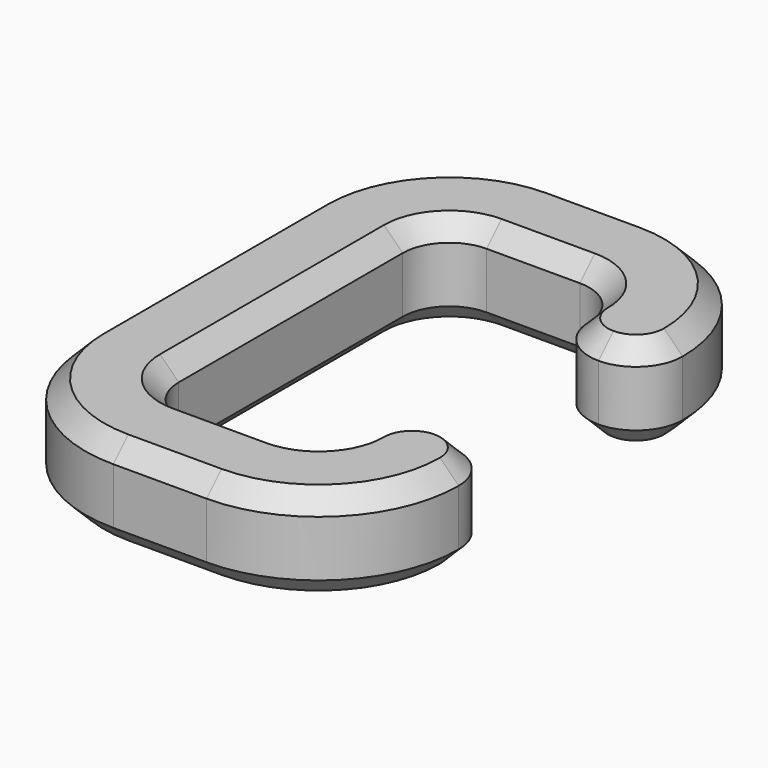
from build123d import *

# Parameters (mm, degrees)
F0_W         = 10
F0_H         = 10
F1_DEPTH     = 10
F2_R         = 4.99999
F3_R         = 15
F4_T1_DEPTH  = 30.00002
F4_T3_DEPTH  = 10
F4_T5_DEPTH  = 1e-05
F4_T7_DEPTH  = 2e-05
F4_T9_DEPTH  = 2e-05
F4_T11_DEPTH = 10.00002
F4_T13_DEPTH = 2e-05
F4_T15_DEPTH = 1e-05
F4_T17_DEPTH = 30
F4_T20_ANGLE = 90
F4_T22_ANGLE = 90
F4_T24_ANGLE = 90
F4_T26_ANGLE = 90
F4_T28_ANGLE = 90
F4_T30_ANGLE = 90
F4_T32_ANGLE = 90
F4_T34_ANGLE = 90
F4_T36_ANGLE = 90
F4_T38_ANGLE = 90
F4_T40_ANGLE = 90
F4_T42_ANGLE = 90
F4_T44_ANGLE = 90
F4_T46_ANGLE = 90
F4_T48_ANGLE = 90
F4_T50_ANGLE = 90
F4_T52_ANGLE = 90
F4_T54_ANGLE = 90
F4_T56_ANGLE = 90
F4_T58_ANGLE = 90
F4_T60_ANGLE = 90
F4_T62_ANGLE = 90
F4_T64_ANGLE = 90
F4_T66_ANGLE = 90


# Not quite as in the source:
# - a fillet or chamfer that OpenCascade refuses, or shapes differently, is made with other operations: its cross-section is extruded or revolved along the edge and cut away or added
# - a fillet or chamfer is up to 0.001 mm smaller than in the source, because OpenCascade refuses the exact size


with BuildPart() as f1:
    # F0 (on Top) → F1 (new body)
    with BuildSketch(Plane.XY):
        Polygon((-10.4597477218, 27.6766866998), (-10.4597477218, 17.6766866998), (-0.4597477218, 17.6766866998), (-0.4597477218, 37.6766866998), (-10.4597477218, 37.6766866998), align=None)
        Polygon((-30.4597477218, 27.6766866998), (-10.4597477218, 27.6766866998), (-10.4597477218, 37.6766866998), (-40.4597477218, 37.6766866998), (-40.4597477218, 27.6766866998), align=None)
        Polygon((-30.4597477218, -12.3233133002), (-30.4597477218, 27.6766866998), (-40.4597477218, 27.6766866998), (-40.4597477218, -22.3233133002), (-30.4597477218, -22.3233133002), align=None)
        Polygon((-10.4597477218, -12.3233133002), (-30.4597477218, -12.3233133002), (-30.4597477218, -22.3233133002), (-0.4597477218, -22.3233133002), (-0.4597477218, -12.3233133002), align=None)
        with Locations((-5.4597477218, -7.3233133002)):
            Rectangle(F0_W, F0_H)
    extrude(amount=F1_DEPTH)

    # F2 (radius 5 in the source; OpenCascade refuses exactly that, so slightly less here)
    f2_edges = [f1.edges().sort_by_distance(p)[0] for p in [
        (-0.459748, 17.676687, 5),
        (-10.459748, 17.676687, 5),
        (-10.459748, 27.676687, 5),
        (-30.459748, 27.676687, 5),
        (-30.459748, -12.323313, 5),
        (-10.459748, -12.323313, 5),
        (-10.459748, -2.323313, 5),
        (-0.459748, -2.323313, 5),
    ]]
    fillet(f2_edges, radius=F2_R)

    # F3
    f3_edges = [f1.edges().sort_by_distance(p)[0] for p in [
        (-0.459748, 37.676687, 5),
        (-40.459748, 37.676687, 5),
        (-0.459748, -22.323313, 5),
        (-40.459748, -22.323313, 5),
    ]]
    fillet(f3_edges, radius=F3_R)

    # F4: chamfer of 2 on 2 edges, made by hand

    # F4_s2 → F4_t1 (cut)
    with BuildSketch(Plane.XZ.offset(-22.6766966998)):
        Polygon((-30.4597477218, 8), (-32.4597477218, 10), (-30.4597477218, 10), align=None)
        Polygon((-32.4597477218, 0), (-30.4597477218, 2), (-30.4597477218, 0), align=None)
    extrude(amount=F4_T1_DEPTH, mode=Mode.SUBTRACT)

    # F4_s4 → F4_t3 (cut)
    with BuildSketch(Plane.YZ.offset(-25.4597477218)):
        Polygon((-20.3233133002, 0), (-22.3233133002, 2), (-22.3233133002, 0), align=None)
        Polygon((35.6766866998, 0), (37.6766866998, 2), (37.6766866998, 0), align=None)
        Polygon((37.6766866998, 8), (35.6766866998, 10), (37.6766866998, 10), align=None)
        Polygon((-22.3233133002, 8), (-20.3233133002, 10), (-22.3233133002, 10), align=None)
    extrude(amount=F4_T3_DEPTH, mode=Mode.SUBTRACT)

    # F4_s6 → F4_t5 (cut)
    with BuildSketch(Plane.XZ.offset(7.3233033002)):
        Polygon((-2.4597477218, 0), (-0.4597477218, 2), (-0.4597477218, 0), align=None)
        Polygon((-0.4597477218, 8), (-2.4597477218, 10), (-0.4597477218, 10), align=None)
    extrude(amount=F4_T5_DEPTH, mode=Mode.SUBTRACT)

    # F4_s8 → F4_t7 (cut)
    with BuildSketch(Plane.YZ.offset(-5.4597577218)):
        Polygon((-4.3233133002, 0), (-2.3233133002, 2), (-2.3233133002, 0), align=None)
        Polygon((19.6766866998, 0), (17.6766866998, 2), (17.6766866998, 0), align=None)
        Polygon((17.6766866998, 8), (19.6766866998, 10), (17.6766866998, 10), align=None)
        Polygon((-2.3233133002, 8), (-4.3233133002, 10), (-2.3233133002, 10), align=None)
    extrude(amount=F4_T7_DEPTH, mode=Mode.SUBTRACT)

    # F4_s10 → F4_t9 (cut)
    with BuildSketch(Plane.XZ.offset(7.3233033002)):
        Polygon((-8.4597477218, 0), (-10.4597477218, 2), (-10.4597477218, 0), align=None)
        Polygon((-10.4597477218, 8), (-8.4597477218, 10), (-10.4597477218, 10), align=None)
    extrude(amount=F4_T9_DEPTH, mode=Mode.SUBTRACT)

    # F4_s12 → F4_t11 (cut)
    with BuildSketch(Plane.YZ.offset(-25.4597577218)):
        Polygon((-14.3233133002, 0), (-12.3233133002, 2), (-12.3233133002, 0), align=None)
        Polygon((29.6766866998, 0), (27.6766866998, 2), (27.6766866998, 0), align=None)
        Polygon((27.6766866998, 8), (29.6766866998, 10), (27.6766866998, 10), align=None)
        Polygon((-12.3233133002, 8), (-14.3233133002, 10), (-12.3233133002, 10), align=None)
    extrude(amount=F4_T11_DEPTH, mode=Mode.SUBTRACT)

    # F4_s14 → F4_t13 (cut)
    with BuildSketch(Plane.XZ.offset(-22.6766966998)):
        Polygon((-8.4597477218, 0), (-10.4597477218, 2), (-10.4597477218, 0), align=None)
        Polygon((-10.4597477218, 8), (-8.4597477218, 10), (-10.4597477218, 10), align=None)
    extrude(amount=F4_T13_DEPTH, mode=Mode.SUBTRACT)

    # F4_s16 → F4_t15 (cut)
    with BuildSketch(Plane.XZ.offset(-22.6766866998)):
        Polygon((-2.4597477218, 0), (-0.4597477218, 2), (-0.4597477218, 0), align=None)
        Polygon((-0.4597477218, 8), (-2.4597477218, 10), (-0.4597477218, 10), align=None)
    extrude(amount=F4_T15_DEPTH, mode=Mode.SUBTRACT)

    # F4_s18 → F4_t17 (cut)
    with BuildSketch(Plane.XZ.offset(-22.6766866998)):
        Polygon((-38.4597477218, 0), (-40.4597477218, 2), (-40.4597477218, 0), align=None)
        Polygon((-40.4597477218, 8), (-38.4597477218, 10), (-40.4597477218, 10), align=None)
    extrude(amount=F4_T17_DEPTH, mode=Mode.SUBTRACT)

    # F4_s19 → F4_t20 (revolve, cut)
    with BuildSketch(Plane.YZ.offset(-15.4597477218)):
        Polygon((-20.3233133002, 0), (-22.3233133002, 2), (-22.3233133002, 0), align=None)
    revolve(axis=Axis((-15.4597477218, -7.3233133002, 0), (0, 0, 1)), revolution_arc=F4_T20_ANGLE, mode=Mode.SUBTRACT)

    # F4_s21 → F4_t22 (revolve, cut)
    with BuildSketch(Plane.XZ.offset(7.3233033002)):
        Polygon((-2.4597477218, 0), (-0.4597477218, 2), (-0.4597477218, 0), align=None)
    revolve(axis=Axis((-5.4597377218, -7.3233033002, 0), (0, 0, 1)), revolution_arc=F4_T22_ANGLE, mode=Mode.SUBTRACT)

    # F4_s23 → F4_t24 (revolve, cut)
    with BuildSketch(Plane.YZ.offset(-5.4597577218)):
        Polygon((-4.3233133002, 0), (-2.3233133002, 2), (-2.3233133002, 0), align=None)
    revolve(axis=Axis((-5.4597577218, -7.3233033002, 0), (0, 0, 1)), revolution_arc=F4_T24_ANGLE, mode=Mode.SUBTRACT)

    # F4_s25 → F4_t26 (revolve, cut)
    with BuildSketch(Plane.XZ.offset(7.3233233002)):
        Polygon((-8.4597477218, 0), (-10.4597477218, 2), (-10.4597477218, 0), align=None)
    revolve(axis=Axis((-15.4597377218, -7.3233233002, 0), (0, 0, -1)), revolution_arc=F4_T26_ANGLE, mode=Mode.SUBTRACT)

    # F4_s27 → F4_t28 (revolve, cut)
    with BuildSketch(Plane.YZ.offset(-25.4597577218)):
        Polygon((-14.3233133002, 0), (-12.3233133002, 2), (-12.3233133002, 0), align=None)
    revolve(axis=Axis((-25.4597577218, -7.3233233002, 0), (0, 0, -1)), revolution_arc=F4_T28_ANGLE, mode=Mode.SUBTRACT)

    # F4_s29 → F4_t30 (revolve, cut)
    with BuildSketch(Plane.XZ.offset(-22.6766966998)):
        Polygon((-32.4597477218, 0), (-30.4597477218, 2), (-30.4597477218, 0), align=None)
    revolve(axis=Axis((-25.4597577218, 22.6766966998, 0), (0, 0, -1)), revolution_arc=F4_T30_ANGLE, mode=Mode.SUBTRACT)

    # F4_s31 → F4_t32 (revolve, cut)
    with BuildSketch(Plane.XZ.offset(-22.6766966998)):
        Polygon((-8.4597477218, 0), (-10.4597477218, 2), (-10.4597477218, 0), align=None)
    revolve(axis=Axis((-15.4597377218, 22.6766966998, 0), (0, 0, 1)), revolution_arc=F4_T32_ANGLE, mode=Mode.SUBTRACT)

    # F4_s33 → F4_t34 (revolve, cut)
    with BuildSketch(Plane.XZ.offset(-22.6766766998)):
        Polygon((-8.4597477218, 0), (-10.4597477218, 2), (-10.4597477218, 0), align=None)
    revolve(axis=Axis((-5.4597577218, 22.6766766998, 0), (0, 0, 1)), revolution_arc=F4_T34_ANGLE, mode=Mode.SUBTRACT)

    # F4_s35 → F4_t36 (revolve, cut)
    with BuildSketch(Plane.YZ.offset(-5.4597377218)):
        Polygon((19.6766866998, 0), (17.6766866998, 2), (17.6766866998, 0), align=None)
    revolve(axis=Axis((-5.4597377218, 22.6766766998, 0), (0, 0, 1)), revolution_arc=F4_T36_ANGLE, mode=Mode.SUBTRACT)

    # F4_s37 → F4_t38 (revolve, cut)
    with BuildSketch(Plane.XZ.offset(-22.6766866998)):
        Polygon((-2.4597477218, 0), (-0.4597477218, 2), (-0.4597477218, 0), align=None)
    revolve(axis=Axis((-15.4597477218, 22.6766866998, 0), (0, 0, 1)), revolution_arc=F4_T38_ANGLE, mode=Mode.SUBTRACT)

    # F4_s39 → F4_t40 (revolve, cut)
    with BuildSketch(Plane.YZ.offset(-25.4597477218)):
        Polygon((35.6766866998, 0), (37.6766866998, 2), (37.6766866998, 0), align=None)
    revolve(axis=Axis((-25.4597477218, 22.6766866998, 0), (0, 0, 1)), revolution_arc=F4_T40_ANGLE, mode=Mode.SUBTRACT)

    # F4_s41 → F4_t42 (revolve, cut)
    with BuildSketch(Plane.XZ.offset(7.3233133002)):
        Polygon((-38.4597477218, 0), (-40.4597477218, 2), (-40.4597477218, 0), align=None)
    revolve(axis=Axis((-25.4597477218, -7.3233133002, 0), (0, 0, 1)), revolution_arc=F4_T42_ANGLE, mode=Mode.SUBTRACT)

    # F4_s43 → F4_t44 (revolve, cut)
    with BuildSketch(Plane.YZ.offset(-25.4597577218)):
        Polygon((-12.3233133002, 8), (-14.3233133002, 10), (-12.3233133002, 10), align=None)
    revolve(axis=Axis((-25.4597577218, -7.3233233002, 10), (0, 0, -1)), revolution_arc=F4_T44_ANGLE, mode=Mode.SUBTRACT)

    # F4_s45 → F4_t46 (revolve, cut)
    with BuildSketch(Plane.XZ.offset(-22.6766966998)):
        Polygon((-30.4597477218, 8), (-32.4597477218, 10), (-30.4597477218, 10), align=None)
    revolve(axis=Axis((-25.4597577218, 22.6766966998, 10), (0, 0, -1)), revolution_arc=F4_T46_ANGLE, mode=Mode.SUBTRACT)

    # F4_s47 → F4_t48 (revolve, cut)
    with BuildSketch(Plane.XZ.offset(-22.6766966998)):
        Polygon((-10.4597477218, 8), (-8.4597477218, 10), (-10.4597477218, 10), align=None)
    revolve(axis=Axis((-15.4597377218, 22.6766966998, 10), (0, 0, 1)), revolution_arc=F4_T48_ANGLE, mode=Mode.SUBTRACT)

    # F4_s49 → F4_t50 (revolve, cut)
    with BuildSketch(Plane.XZ.offset(-22.6766766998)):
        Polygon((-10.4597477218, 8), (-8.4597477218, 10), (-10.4597477218, 10), align=None)
    revolve(axis=Axis((-5.4597577218, 22.6766766998, 10), (0, 0, 1)), revolution_arc=F4_T50_ANGLE, mode=Mode.SUBTRACT)

    # F4_s51 → F4_t52 (revolve, cut)
    with BuildSketch(Plane.YZ.offset(-5.4597377218)):
        Polygon((17.6766866998, 8), (19.6766866998, 10), (17.6766866998, 10), align=None)
    revolve(axis=Axis((-5.4597377218, 22.6766766998, 10), (0, 0, 1)), revolution_arc=F4_T52_ANGLE, mode=Mode.SUBTRACT)

    # F4_s53 → F4_t54 (revolve, cut)
    with BuildSketch(Plane.XZ.offset(-22.6766866998)):
        Polygon((-0.4597477218, 8), (-2.4597477218, 10), (-0.4597477218, 10), align=None)
    revolve(axis=Axis((-15.4597477218, 22.6766866998, 10), (0, 0, 1)), revolution_arc=F4_T54_ANGLE, mode=Mode.SUBTRACT)

    # F4_s55 → F4_t56 (revolve, cut)
    with BuildSketch(Plane.YZ.offset(-25.4597477218)):
        Polygon((37.6766866998, 8), (35.6766866998, 10), (37.6766866998, 10), align=None)
    revolve(axis=Axis((-25.4597477218, 22.6766866998, 10), (0, 0, 1)), revolution_arc=F4_T56_ANGLE, mode=Mode.SUBTRACT)

    # F4_s57 → F4_t58 (revolve, cut)
    with BuildSketch(Plane.XZ.offset(7.3233133002)):
        Polygon((-40.4597477218, 8), (-38.4597477218, 10), (-40.4597477218, 10), align=None)
    revolve(axis=Axis((-25.4597477218, -7.3233133002, 10), (0, 0, 1)), revolution_arc=F4_T58_ANGLE, mode=Mode.SUBTRACT)

    # F4_s59 → F4_t60 (revolve, cut)
    with BuildSketch(Plane.YZ.offset(-15.4597477218)):
        Polygon((-22.3233133002, 8), (-20.3233133002, 10), (-22.3233133002, 10), align=None)
    revolve(axis=Axis((-15.4597477218, -7.3233133002, 10), (0, 0, 1)), revolution_arc=F4_T60_ANGLE, mode=Mode.SUBTRACT)

    # F4_s61 → F4_t62 (revolve, cut)
    with BuildSketch(Plane.XZ.offset(7.3233033002)):
        Polygon((-0.4597477218, 8), (-2.4597477218, 10), (-0.4597477218, 10), align=None)
    revolve(axis=Axis((-5.4597377218, -7.3233033002, 10), (0, 0, 1)), revolution_arc=F4_T62_ANGLE, mode=Mode.SUBTRACT)

    # F4_s63 → F4_t64 (revolve, cut)
    with BuildSketch(Plane.YZ.offset(-5.4597577218)):
        Polygon((-2.3233133002, 8), (-4.3233133002, 10), (-2.3233133002, 10), align=None)
    revolve(axis=Axis((-5.4597577218, -7.3233033002, 10), (0, 0, 1)), revolution_arc=F4_T64_ANGLE, mode=Mode.SUBTRACT)

    # F4_s65 → F4_t66 (revolve, cut)
    with BuildSketch(Plane.XZ.offset(7.3233233002)):
        Polygon((-10.4597477218, 8), (-8.4597477218, 10), (-10.4597477218, 10), align=None)
    revolve(axis=Axis((-15.4597377218, -7.3233233002, 10), (0, 0, -1)), revolution_arc=F4_T66_ANGLE, mode=Mode.SUBTRACT)


solid = f1.part
